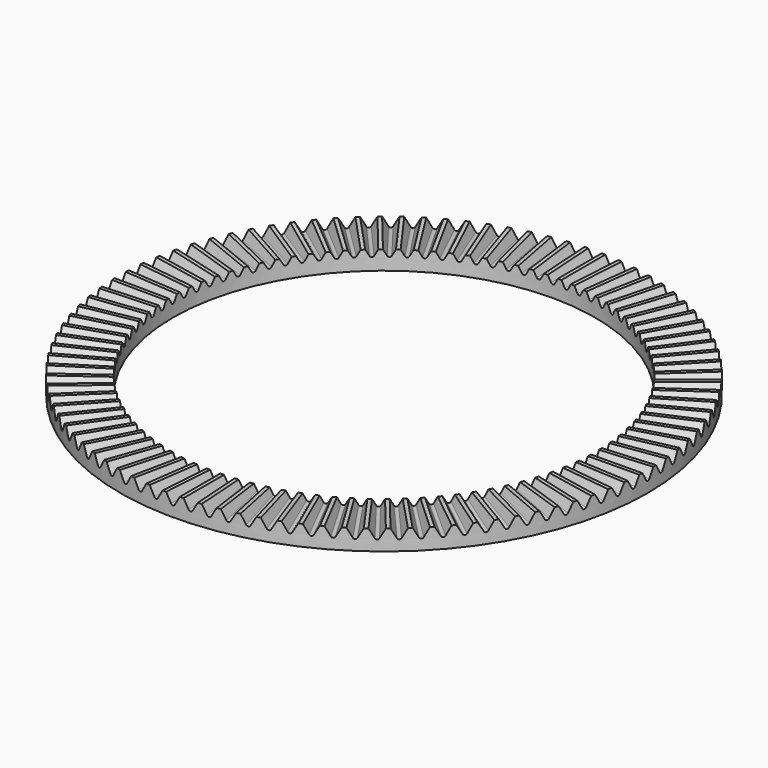
from build123d import *

# Parameters (mm, degrees)
F11_COPIES_COUNT = 96


# Not quite as in the source:
# - a pattern or mirror of a feature is missing from the dataset's text; its kind, count and spacing are read off the source's solid


with BuildPart() as f10:
    # F7 (on Front) → F10 (revolve)
    with BuildSketch(Plane.XZ):
        Polygon((250, 10.4666947111), (200, 9.0489679152), (200, 2.7088633979), (200, -8.7088633979), (250, -8.7088633979), (250, 1.2911366021), align=None)
    revolve(axis=Axis((0, 0, 6.3789156566), (0, 0, 1)))

    # F11: sweep along a path in F9
    with BuildLine(Plane.XZ) as f11_path:
        Line((250, 1.2911366021), (195.0020087381, 2.8505791207))
    # F8 (on offset) → F11 (sweep, cut)
    with BuildSketch(Plane.YZ.offset(250)):
        with BuildLine():
            Line((1.7320508076, 2.2911366021), (6.4522114826, 10.4666947111))
            Line((6.4522114826, 10.4666947111), (-6.4522114826, 10.4666947111))
            Line((-6.4522114826, 10.4666947111), (-1.7320508076, 2.2911366021))
            ThreePointArc((-1.7320508076, 2.2911366021), (0, 1.2911366021), (1.7320508076, 2.2911366021))
        make_face()
    f11 = sweep(path=f11_path.line, mode=Mode.SUBTRACT)

    # F11_copies: F11 ×96 about axis
    f11_copies_axis = Axis((0, 0, 0), (0, 0, 1))
    for i in range(1, F11_COPIES_COUNT):
        add(f11.rotate(f11_copies_axis, i * 360 / F11_COPIES_COUNT), mode=Mode.SUBTRACT)


solid = f10.part
